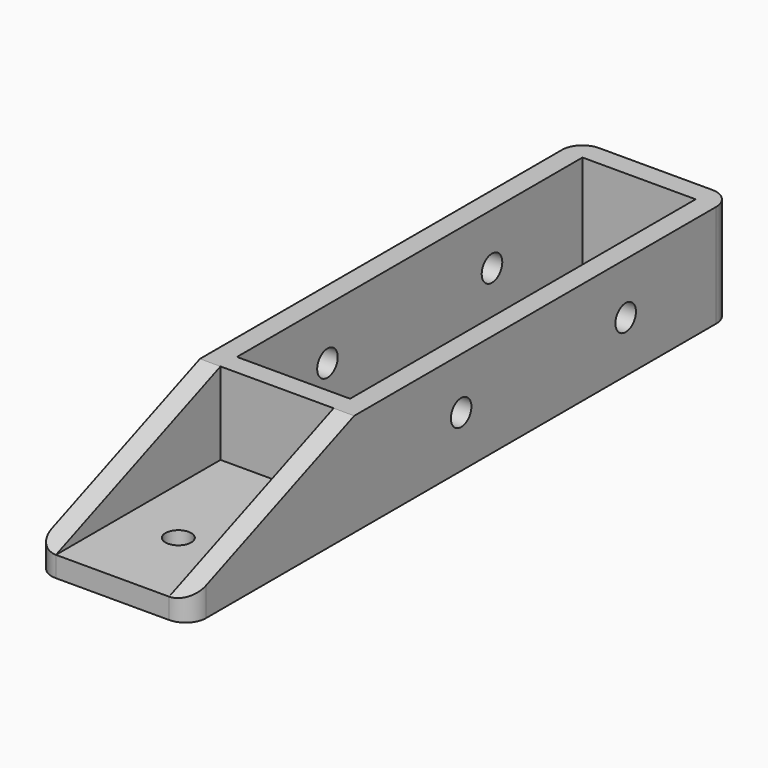
from build123d import *

# Parameters (mm, degrees)
F0_W      = 11
F0_H      = 42
F1_DEPTH  = 10
F2_T      = 2
F3_W      = 15
F3_H      = 20
F4_DEPTH  = 2
F6_DEPTH  = 2
F8_R      = 1.25
F9_DEPTH  = 2.001
F10_R     = 1.25
F11_DEPTH = 15.001
F12_R     = 2


# Not quite as in the source:
# - a pattern or mirror of a feature is missing from the dataset's text; its kind, count and spacing are read off the source's solid


with BuildPart() as f1:
    # F0 (on Top) → F1 (new body)
    with BuildSketch(Plane.XY):
        with Locations((5.5, 21)):
            Rectangle(F0_W, F0_H)
    extrude(amount=F1_DEPTH)

    # F2
    f2_openings = [f1.faces().sort_by_distance(p)[0] for p in [
        (5.5, 21, 10),
        (5.5, 21, 0),
    ]]
    offset(amount=F2_T, openings=f2_openings, kind=Kind.INTERSECTION)

    # F3 (on Top) → F4 (join)
    with BuildSketch(Plane.XY):
        with Locations((5.5, -12)):
            Rectangle(F3_W, F3_H)
    extrude(amount=F4_DEPTH)

    # F5 (on face) → F6 (join)
    with BuildSketch(Plane.YZ.offset(13)):
        Polygon((-2, 10), (-22, 2), (-2, 2), align=None)
    f6 = extrude(amount=-F6_DEPTH)

    # F6_copies: F6 across plane
    add(f6.mirror(Plane(origin=(5.5, 0, 0), x_dir=(0, 0, -1), z_dir=(-1, 0, 0))))

    # F8 (on face) → F9 (cut, through all)
    with BuildSketch(Plane.XY.offset(2)):
        with Locations((5.5, -14)):
            Circle(F8_R)
    extrude(amount=-F9_DEPTH, mode=Mode.SUBTRACT)

    # F10 (on face) → F11 (cut, through all)
    with BuildSketch(Plane.YZ.offset(13)):
        with Locations((11, 5)):
            Circle(F10_R)
        with Locations((31, 5)):
            Circle(F10_R)
    extrude(amount=-F11_DEPTH, mode=Mode.SUBTRACT)

    # F12
    f12_edges = [f1.edges().sort_by_distance(p)[0] for p in [
        (-2, -22, 1),
        (13, -22, 1),
        (13, 44, 5),
        (-2, 44, 5),
    ]]
    fillet(f12_edges, radius=F12_R)


solid = f1.part
